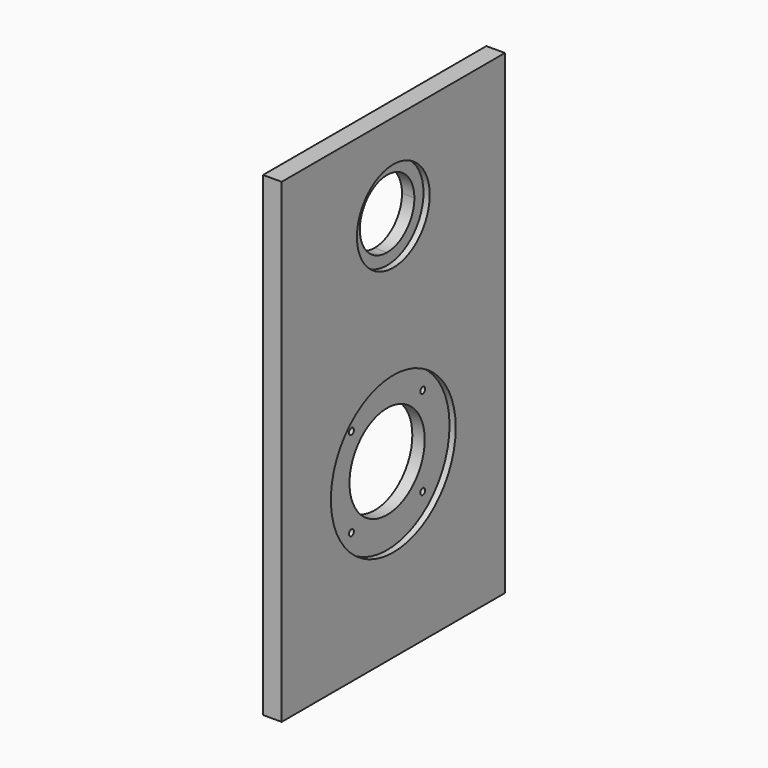
from build123d import *

# Parameters (mm, degrees)
F1_DEPTH = 9
F0_R     = 1.5
F2_DEPTH = 6


# Not quite as in the source:
# - a feature names something its author has since deleted; it is built from what else it names


with BuildPart() as f1:
    # F0 (on Right) → F1 (new body)
    with BuildSketch(Plane.YZ):
        with BuildLine():
            Line((0, 115), (-67.5, 115))
            Line((-67.5, 115), (-67.5, -115))
            Line((-67.5, -115), (0, -115))
            Line((0, -115), (0, -70.25))
            ThreePointArc((0, -70.25), (-37.75, -32.5), (0, 5.25))
            Line((0, 5.25), (0, 51))
            ThreePointArc((0, 51), (-22, 73), (0, 95))
            Line((0, 95), (0, 115))
        make_face()
        with BuildLine():
            Line((67.5, 115), (0, 115))
            Line((0, 115), (0, 95))
            ThreePointArc((0, 95), (15.5563491861, 88.5563491861), (22, 73))
            ThreePointArc((22, 73), (15.5563491861, 57.4436508139), (0, 51))
            Line((0, 51), (0, 5.25))
            ThreePointArc((0, 5.25), (26.6932809898, -5.8067190102), (37.75, -32.5))
            ThreePointArc((37.75, -32.5), (26.6932809898, -59.1932809898), (0, -70.25))
            Line((0, -70.25), (0, -115))
            Line((0, -115), (67.5, -115))
            Line((67.5, -115), (67.5, 115))
        make_face()
    extrude(amount=F1_DEPTH)

    # F0 (on Right) → F2 (join)
    with BuildSketch(Plane.YZ):
        with BuildLine():
            Line((0, 89.5), (0, 95))
            ThreePointArc((0, 95), (-22, 73), (0, 51))
            Line((0, 51), (0, 56.5))
            ThreePointArc((0, 56.5), (-16.5, 73), (0, 89.5))
        make_face()
        with BuildLine():
            ThreePointArc((22, 73), (15.5563491861, 88.5563491861), (0, 95))
            Line((0, 95), (0, 89.5))
            ThreePointArc((0, 89.5), (11.6672618896, 84.6672618896), (16.5, 73))
            ThreePointArc((16.5, 73), (11.6672618896, 61.3327381104), (0, 56.5))
            Line((0, 56.5), (0, 51))
            ThreePointArc((0, 51), (15.5563491861, 57.4436508139), (22, 73))
        make_face()
        with BuildLine():
            ThreePointArc((0, 5.25), (-37.75, -32.5), (0, -70.25))
            Line((0, -70.25), (0, -55.25))
            ThreePointArc((0, -55.25), (-22.75, -32.5), (0, -9.75))
            Line((0, -9.75), (0, 5.25))
        make_face()
        with Locations((-21.5667568262, -54.0667568262)):
            Circle(F0_R, mode=Mode.SUBTRACT)
        with Locations((-21.5667568262, -10.9332431738)):
            Circle(F0_R, mode=Mode.SUBTRACT)
        with BuildLine():
            Line((0, -55.25), (0, -70.25))
            ThreePointArc((0, -70.25), (26.6932809898, -59.1932809898), (37.75, -32.5))
            ThreePointArc((37.75, -32.5), (26.6932809898, -5.8067190102), (0, 5.25))
            Line((0, 5.25), (0, -9.75))
            ThreePointArc((0, -9.75), (16.086679272, -16.413320728), (22.75, -32.5))
            ThreePointArc((22.75, -32.5), (16.086679272, -48.586679272), (0, -55.25))
        make_face()
        with Locations((21.5667568262, -54.0667568262)):
            Circle(F0_R, mode=Mode.SUBTRACT)
        with Locations((21.5667568262, -10.9332431738)):
            Circle(F0_R, mode=Mode.SUBTRACT)
    extrude(amount=F2_DEPTH)


solid = f1.part
